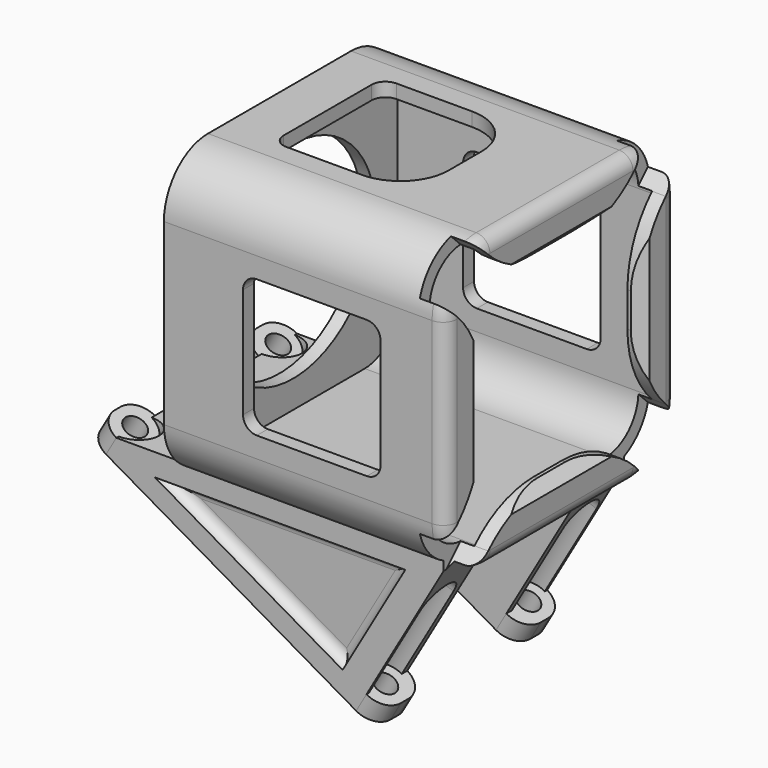
from build123d import *

# Parameters (mm, degrees)
F1_DEPTH      = 18.5
F3_DEPTH      = 2
F4_SIZE       = 1.5
F6_DEPTH      = 5
F7_W          = 39
F7_H          = 14
F8_DEPTH      = 25
F10_DEPTH     = 22.5
F11_R         = 15
F12_DEPTH     = 2
F14_DEPTH     = 16.42
F16_W         = 3
F16_H         = 18.84
F17_DEPTH     = 3.5
F18_R         = 2.99999
F20_DEPTH     = 9
F21_R         = 3
F15_R         = 1.6
F22_DEPTH     = 12.5
F23_R         = 3
F24_DEPTH     = 15
F26_DEPTH     = 25
F27_R         = 2
F28_R         = 15.25
F29_R         = 3
F31_DEPTH     = 2
F33_START     = 15
F33_DEPTH     = 2
F34_START     = -15
F34_DEPTH     = 2
F35_T1_DEPTH  = 21.9518391761
F35_T3_DEPTH  = 35.2804172955
F35_T8_DEPTH  = 43.9036783522
F35_T13_DEPTH = 43.9036783522


# Not quite as in the source:
# - a fillet or chamfer that OpenCascade refuses, or shapes differently, is made with other operations: its cross-section is extruded or revolved along the edge and cut away or added
# - a fillet or chamfer is up to 0.001 mm smaller than in the source, because OpenCascade refuses the exact size


with BuildPart() as f1:
    # F0 (on Right) → F1 (new body, symmetric)
    with BuildSketch(Plane.YZ):
        with BuildLine():
            Line((13, 21), (-13, 21))
            ThreePointArc((-13, 21), (-18.6568542495, 18.6568542495), (-21, 13))
            Line((-21, 13), (-21, -13))
            ThreePointArc((-21, -13), (-18.6568542495, -18.6568542495), (-13, -21))
            Line((-13, -21), (13, -21))
            ThreePointArc((13, -21), (18.6568542495, -18.6568542495), (21, -13))
            Line((21, -13), (21, 13))
            ThreePointArc((21, 13), (18.6568542495, 18.6568542495), (13, 21))
        make_face()
        with BuildLine():
            ThreePointArc((-19, 13), (-17.2426406871, 17.2426406871), (-13, 19))
            Line((-13, 19), (13, 19))
            ThreePointArc((13, 19), (17.2426406871, 17.2426406871), (19, 13))
            Line((19, 13), (19, -13))
            ThreePointArc((19, -13), (17.2426406871, -17.2426406871), (13, -19))
            Line((13, -19), (-13, -19))
            ThreePointArc((-13, -19), (-17.2426406871, -17.2426406871), (-19, -13))
            Line((-19, -13), (-19, 13))
        make_face(mode=Mode.SUBTRACT)
    extrude(amount=F1_DEPTH, both=True)

    # F2 (on face) → F3 (join)
    with BuildSketch(Plane.YZ.offset(18.5)):
        with BuildLine():
            Line((13, 21), (-13, 21))
            ThreePointArc((-13, 21), (-18.6568542495, 18.6568542495), (-21, 13))
            Line((-21, 13), (-21, -13))
            ThreePointArc((-21, -13), (-18.6568542495, -18.6568542495), (-13, -21))
            Line((-13, -21), (13, -21))
            ThreePointArc((13, -21), (18.6568542495, -18.6568542495), (21, -13))
            Line((21, -13), (21, 13))
            ThreePointArc((21, 13), (18.6568542495, 18.6568542495), (13, 21))
        make_face()
        with BuildLine():
            ThreePointArc((-14.5, 12.5), (-13.9142135624, 13.9142135624), (-12.5, 14.5))
            Line((-12.5, 14.5), (12.5, 14.5))
            ThreePointArc((12.5, 14.5), (13.9142135624, 13.9142135624), (14.5, 12.5))
            Line((14.5, 12.5), (14.5, -12.5))
            ThreePointArc((14.5, -12.5), (13.9142135624, -13.9142135624), (12.5, -14.5))
            Line((12.5, -14.5), (-12.5, -14.5))
            ThreePointArc((-12.5, -14.5), (-13.9142135624, -13.9142135624), (-14.5, -12.5))
            Line((-14.5, -12.5), (-14.5, 12.5))
        make_face(mode=Mode.SUBTRACT)
    extrude(amount=F3_DEPTH)

    # F4
    f4_edges = [f1.edges().sort_by_distance(p)[0] for p in [
        (20.5, 0, 14.5),
    ]]
    chamfer(f4_edges, length=F4_SIZE)

    # F5 (on face) → F6 (cut)
    with BuildSketch(Plane.XY.offset(21)):
        with BuildLine():
            Line((-0.5, 10), (-11.5, 10))
            ThreePointArc((-11.5, 10), (-12.9142135624, 9.4142135624), (-13.5, 8))
            Line((-13.5, 8), (-13.5, -8))
            ThreePointArc((-13.5, -8), (-12.9142135624, -9.4142135624), (-11.5, -10))
            Line((-11.5, -10), (-0.5, -10))
            ThreePointArc((-0.5, -10), (4.4497474683, -7.9497474683), (6.5, -3))
            Line((6.5, -3), (6.5, 3))
            ThreePointArc((6.5, 3), (4.4497474683, 7.9497474683), (-0.5, 10))
        make_face()
    extrude(amount=-F6_DEPTH, mode=Mode.SUBTRACT)

    # F7 (on face) → F8 (cut)
    with BuildSketch(Plane(origin=(0, 0, -21), x_dir=(1, 0, 0), z_dir=(0, 0, -1))):
        with Locations((1, 0)):
            Rectangle(F7_W, F7_H)
    extrude(amount=F8_DEPTH, mode=Mode.SUBTRACT)

    # F9 (on Front) → F10 (cut, symmetric)
    with BuildSketch(Plane.XZ):
        with BuildLine():
            ThreePointArc((11, 8), (10.4142135624, 9.4142135624), (9, 10))
            Line((9, 10), (-7, 10))
            ThreePointArc((-7, 10), (-8.4142135624, 9.4142135624), (-9, 8))
            Line((-9, 8), (-9, -8))
            ThreePointArc((-9, -8), (-8.4142135624, -9.4142135624), (-7, -10))
            Line((-7, -10), (9, -10))
            ThreePointArc((9, -10), (10.4142135624, -9.4142135624), (11, -8))
            Line((11, -8), (11, 8))
        make_face()
    extrude(amount=F10_DEPTH, both=True, mode=Mode.SUBTRACT)

    # F11 (on face) → F12 (join)
    with BuildSketch(Plane(origin=(-18.5, 0, 0), x_dir=(0, -1, 0), z_dir=(-1, 0, 0))):
        with BuildLine():
            Line((13, 21), (-13, 21))
            ThreePointArc((-13, 21), (-18.6568542495, 18.6568542495), (-21, 13))
            Line((-21, 13), (-21, -13))
            ThreePointArc((-21, -13), (-18.6568542495, -18.6568542495), (-13, -21))
            Line((-13, -21), (13, -21))
            ThreePointArc((13, -21), (18.6568542495, -18.6568542495), (21, -13))
            Line((21, -13), (21, 13))
            ThreePointArc((21, 13), (18.6568542495, 18.6568542495), (13, 21))
        make_face()
        Circle(F11_R, mode=Mode.SUBTRACT)
    extrude(amount=F12_DEPTH)

    # F13 (on Front) → F14 (join, symmetric)
    with BuildSketch(Plane.XZ):
        Polygon((6.3886946446, -45.0980762114), (7.8886946446, -42.5), (5.2906184332, -41), (17.4149740862, -20), (-20.5, -20), (-31.0824485257, -20), (-33.6805247371, -18.5), (-35.1805247371, -21.0980762114), align=None)
    extrude(amount=F14_DEPTH, both=True)

    # F16 (on face) → F17 (cut)
    with BuildSketch(Plane(origin=(-17.9308661693, 0, -31.0571712289), x_dir=(0.8660254038, 0, -0.5), z_dir=(-0.5, 0, -0.8660254038))):
        with Locations((-18.4181900351, 0)):
            Rectangle(F16_W, F16_H)
    extrude(amount=-F17_DEPTH, mode=Mode.SUBTRACT)

    # F18 (radius 3 in the source; OpenCascade refuses exactly that, so slightly less here)
    f18_edges = [f1.edges().sort_by_distance(p)[0] for p in [
        (-34.430525, 16.42, -19.799038),
        (-34.430525, 9.42, -19.799038),
        (-34.430525, -9.42, -19.799038),
        (-34.430525, -16.42, -19.799038),
    ]]
    fillet(f18_edges, radius=F18_R)

    # F19 (on Front) → F20 (cut, symmetric)
    with BuildSketch(Plane.XZ):
        Polygon((-10.9318134311, -35.0980762114), (6.3886946446, -45.0980762114), (20.3017254322, -21), (-2.7922853354, -21), align=None)
    extrude(amount=F20_DEPTH, both=True, mode=Mode.SUBTRACT)

    # F21
    f21_edges = [f1.edges().sort_by_distance(p)[0] for p in [
        (-6.862049, 9, -28.049038),
        (-6.862049, -9, -28.049038),
    ]]
    fillet(f21_edges, radius=F21_R)

    # F15 (on face) → F22 (cut, symmetric)
    with BuildSketch(Plane(origin=(-16.4308661693, 0, -28.4590950176), x_dir=(0.8660254038, 0, -0.5), z_dir=(0.5, 0, 0.8660254038))):
        with Locations((25.0818099649, -13)):
            Circle(F15_R)
        with Locations((25.0818099649, 13)):
            Circle(F15_R)
        with Locations((-16.9181900351, -13)):
            Circle(F15_R)
        with Locations((-16.9181900351, 13)):
            Circle(F15_R)
    extrude(amount=F22_DEPTH, both=True, mode=Mode.SUBTRACT)

    # F23 (on face) → F24 (cut)
    with BuildSketch(Plane(origin=(-16.4308661693, 0, -28.4590950176), x_dir=(0.8660254038, 0, -0.5), z_dir=(0.5, 0, 0.8660254038))):
        with Locations((-16.9181900351, -13)):
            Circle(F23_R)
        with Locations((25.0818099649, -13)):
            Circle(F23_R)
        with Locations((-16.9181900351, 13)):
            Circle(F23_R)
        with Locations((25.0818099649, 13)):
            Circle(F23_R)
    extrude(amount=F24_DEPTH, mode=Mode.SUBTRACT)

    # F25 (on face) → F26 (cut)
    with BuildSketch(Plane(origin=(18.5, 0, 0), x_dir=(0, -1, 0), z_dir=(-1, 0, 0))):
        with BuildLine():
            ThreePointArc((-16.4102058828, 22.0670601323), (-19.4454364826, 19.4454364826), (-22.0670601323, 16.4102058828))
            Line((-22.0670601323, 16.4102058828), (-5.6568542495, 0))
            Line((-5.6568542495, 0), (-22.0670601323, -16.4102058828))
            ThreePointArc((-22.0670601323, -16.4102058828), (-19.4454364826, -19.4454364826), (-16.4102058828, -22.0670601323))
            Line((-16.4102058828, -22.0670601323), (0, -5.6568542495))
            Line((0, -5.6568542495), (16.4102058828, -22.0670601323))
            ThreePointArc((16.4102058828, -22.0670601323), (19.4454364826, -19.4454364826), (22.0670601323, -16.4102058828))
            Line((22.0670601323, -16.4102058828), (5.6568542495, 0))
            Line((5.6568542495, 0), (22.0670601323, 16.4102058828))
            ThreePointArc((22.0670601323, 16.4102058828), (19.4454364826, 19.4454364826), (16.4102058828, 22.0670601323))
            Line((16.4102058828, 22.0670601323), (0, 5.6568542495))
            Line((0, 5.6568542495), (-16.4102058828, 22.0670601323))
        make_face()
    extrude(amount=-F26_DEPTH, mode=Mode.SUBTRACT)

    # F27
    f27_edges = [f1.edges().sort_by_distance(p)[0] for p in [
        (20.5, 0, 21),
        (20.5, -21, 0),
        (20.5, 21, 0),
        (20.5, 0, -21),
        (20.5, -20.931559, -14.04421),
        (20.5, -14.04421, -20.931559),
        (20.5, 14.04421, -20.931559),
        (20.5, 20.931559, -14.04421),
        (20.5, -14.04421, 20.931559),
        (20.5, -20.931559, 14.04421),
        (20.5, 20.931559, 14.04421),
        (20.5, 14.04421, 20.931559),
    ]]
    fillet(f27_edges, radius=F27_R)

    # F28
    f28_edges = [f1.edges().sort_by_distance(p)[0] for p in [
        (18.75, -14.5, 8.843146),
        (18.75, -8.843146, 14.5),
        (18.75, 8.843146, 14.5),
        (18.75, 14.5, 8.843146),
        (18.75, 14.5, -8.843146),
        (18.75, 8.843146, -14.5),
        (18.75, -14.5, -8.843146),
        (18.75, -8.843146, -14.5),
    ]]
    fillet(f28_edges, radius=F28_R)

    # F29
    f29_edges = [f1.edges().sort_by_distance(p)[0] for p in [
        (7.138695, -16.42, -43.799038),
        (7.138695, -9, -43.799038),
        (7.138695, 9, -43.799038),
        (7.138695, 16.42, -43.799038),
    ]]
    fillet(f29_edges, radius=F29_R)

    # F24_face (on face) → F30 (revolve, cut)
    with BuildSketch(Plane(origin=(11.6879606424, -13, -27.3729991709), x_dir=(0, -1, 0), z_dir=(-0.5, 0, -0.8660254038))):
        with BuildLine():
            Line((-3, -1.2732395447), (3, -1.2732395447))
            ThreePointArc((3, -1.2732395447), (0, 1.7267604553), (-3, -1.2732395447))
        make_face()
        with BuildLine():
            Line((-29, -1.2732395447), (-23, -1.2732395447))
            ThreePointArc((-23, -1.2732395447), (-26, 1.7267604553), (-29, -1.2732395447))
        make_face()
    revolve(axis=Axis((12.7906184332, -13, -28.0096189432), (0, -1, 0)), mode=Mode.SUBTRACT)

    # F25 (on face) → F31 (cut)
    with BuildSketch(Plane(origin=(18.5, 0, 0), x_dir=(0, -1, 0), z_dir=(-1, 0, 0))):
        with BuildLine():
            ThreePointArc((-16.4102058828, 22.0670601323), (-19.4454364826, 19.4454364826), (-22.0670601323, 16.4102058828))
            Line((-22.0670601323, 16.4102058828), (-5.6568542495, 0))
            Line((-5.6568542495, 0), (-22.0670601323, -16.4102058828))
            ThreePointArc((-22.0670601323, -16.4102058828), (-19.4454364826, -19.4454364826), (-16.4102058828, -22.0670601323))
            Line((-16.4102058828, -22.0670601323), (0, -5.6568542495))
            Line((0, -5.6568542495), (16.4102058828, -22.0670601323))
            ThreePointArc((16.4102058828, -22.0670601323), (19.4454364826, -19.4454364826), (22.0670601323, -16.4102058828))
            Line((22.0670601323, -16.4102058828), (5.6568542495, 0))
            Line((5.6568542495, 0), (22.0670601323, 16.4102058828))
            ThreePointArc((22.0670601323, 16.4102058828), (19.4454364826, 19.4454364826), (16.4102058828, 22.0670601323))
            Line((16.4102058828, 22.0670601323), (0, 5.6568542495))
            Line((0, 5.6568542495), (-16.4102058828, 22.0670601323))
        make_face()
    extrude(amount=F31_DEPTH, mode=Mode.SUBTRACT)

    # F32 (on Front) → F33 (cut)
    with BuildSketch(Plane.XZ.offset(F33_START)):
        Polygon((1.8265168181, -39), (10.9301049718, -23.2321227866), (-25.4842476431, -23.2321227866), align=None)
    extrude(amount=F33_DEPTH, mode=Mode.SUBTRACT)

    # F32 (on Front) → F34 (cut)
    with BuildSketch(Plane.XZ.offset(F34_START)):
        Polygon((1.8265168181, -39), (10.9301049718, -23.2321227866), (-25.4842476431, -23.2321227866), align=None)
    extrude(amount=-F34_DEPTH, mode=Mode.SUBTRACT)

    # F35: fillet of radius 1.5 on 6 edges, made by hand

    # F35_s2 → F35_t1 (join)
    with BuildSketch(Plane(origin=(-16.4308661693, 0, -28.4590950176), x_dir=(0, 1, 0), z_dir=(0.5, 0, 0.8660254038))):
        with BuildLine():
            ThreePointArc((16.42, -21.0818099649), (15.4114229471, -20.6159331895), (15, -19.5839448174))
            Line((15, -19.5839448174), (15, -21.0818099649))
            Line((15, -21.0818099649), (16.42, -21.0818099649))
        make_face()
        with BuildLine():
            ThreePointArc((-16.42, -21.0818099649), (-15.4114229471, -20.6159331895), (-15, -19.5839448174))
            Line((-15, -19.5839448174), (-15, -21.0818099649))
            Line((-15, -21.0818099649), (-16.42, -21.0818099649))
        make_face()
    extrude(amount=F35_T1_DEPTH)

    # F35_s4 → F35_t3 (join)
    with BuildSketch(Plane(origin=(-12.2963546467, 0, 7.0993036653), x_dir=(0, 1, 0), z_dir=(0.8660254038, 0, -0.5))):
        with BuildLine():
            ThreePointArc((16.42, -32.8617323386), (15.4114229471, -32.3958555631), (15, -31.3638671911))
            Line((15, -31.3638671911), (15, -32.8617323386))
            Line((15, -32.8617323386), (16.42, -32.8617323386))
        make_face()
        with BuildLine():
            ThreePointArc((-16.42, -32.8617323386), (-15.4114229471, -32.3958555631), (-15, -31.3638671911))
            Line((-15, -31.3638671911), (-15, -32.8617323386))
            Line((-15, -32.8617323386), (-16.42, -32.8617323386))
        make_face()
    extrude(amount=F35_T3_DEPTH)


with BuildPart() as f35_tool6:
    # F35_s7 → F35_t8 (new body)
    with BuildSketch(Plane.YZ.offset(14.6747678405)):
        with BuildLine():
            ThreePointArc((16.42, -23.2321227866), (15.4114229471, -23.697999562), (15, -24.729987934))
            Line((15, -24.729987934), (15, -23.2321227866))
            Line((15, -23.2321227866), (16.42, -23.2321227866))
        make_face()
    extrude(amount=-F35_T8_DEPTH)

    split(bisect_by=Plane(origin=(-16.4308661693, 0, -28.4590950176), x_dir=(0, 1, 0), z_dir=(0.5, 0, 0.8660254038)), keep=Keep.TOP)


with BuildPart() as f1_1:
    add(f1.part)

    # F35_t5: union F35_tool6
    add(f35_tool6.part)


with BuildPart() as f35_tool11:
    # F35_s12 → F35_t13 (new body)
    with BuildSketch(Plane.YZ.offset(14.6747678405)):
        with BuildLine():
            ThreePointArc((-16.42, -23.2321227866), (-15.4114229471, -23.697999562), (-15, -24.729987934))
            Line((-15, -24.729987934), (-15, -23.2321227866))
            Line((-15, -23.2321227866), (-16.42, -23.2321227866))
        make_face()
    extrude(amount=-F35_T13_DEPTH)

    split(bisect_by=Plane(origin=(-16.4308661693, 0, -28.4590950176), x_dir=(0, 1, 0), z_dir=(0.5, 0, 0.8660254038)), keep=Keep.TOP)


with BuildPart() as f1_2:
    add(f1_1.part)

    # F35_t10: union F35_tool11
    add(f35_tool11.part)


solid = f1_2.part
